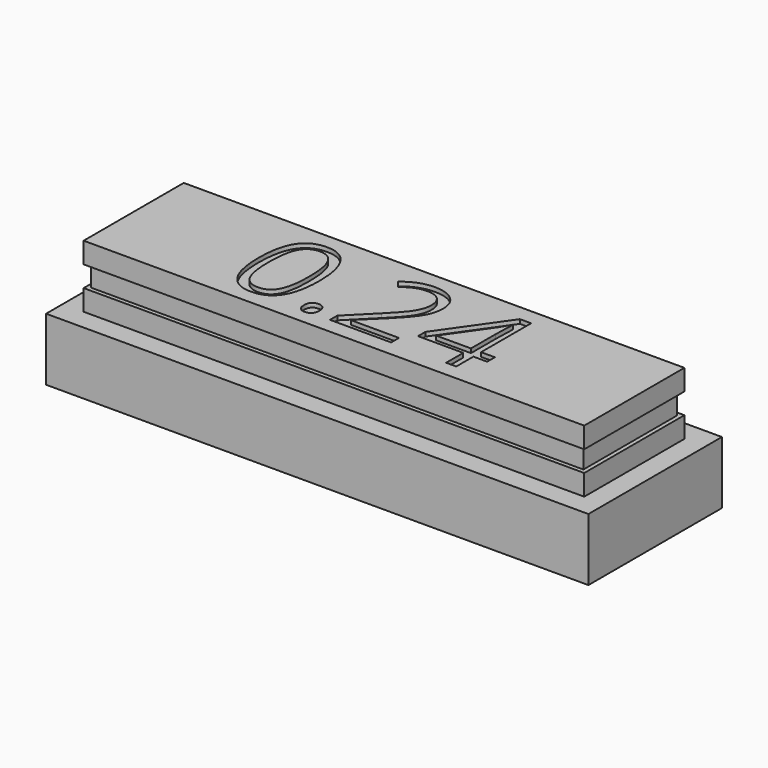
from build123d import *

# Parameters (mm, degrees)
F0_W         = 26
F0_H         = 8
F0_W_2       = 20
F0_H_2       = 2
F1_DEPTH     = 3
F2_W         = 24
F2_H         = 6
F3_DEPTH     = 3
F5_W         = 24
F5_H         = 6
F5_W_2       = 23.6
F5_H_2       = 5.6
F6_DEPTH     = 0.5
F7_W         = 19.52
F7_H         = 1.52
F8_DEPTH     = 3
F9_TEXT_SIZE = 6.25
F10_DEPTH    = 0.2


# Not quite as in the source:
# - Text() gives the source's letters only with a copy of the font that has no kerning and outlines rounded to 1/6400 em; it was checked with that copy


with BuildPart() as f1:
    # F0 (on Top) → F1 (new body)
    with BuildSketch(Plane.XY):
        Rectangle(F0_W, F0_H)
        Rectangle(F0_W_2, F0_H_2, mode=Mode.SUBTRACT)
    extrude(amount=F1_DEPTH)


with BuildPart() as f3:
    # F2 (on face) → F3 (new body)
    with BuildSketch(Plane.XY.offset(3)):
        Rectangle(F2_W, F2_H)
    extrude(amount=F3_DEPTH)

    # F5 (on mid) → F6 (cut, symmetric)
    with BuildSketch(Plane.XY.offset(4.5)):
        Rectangle(F5_W, F5_H)
        Rectangle(F5_W_2, F5_H_2, mode=Mode.SUBTRACT)
    extrude(amount=F6_DEPTH, both=True, mode=Mode.SUBTRACT)

    # F7 (on face) → F8 (join, through all)
    with BuildSketch(Plane(origin=(0, 0, 3), x_dir=(1, 0, 0), z_dir=(0, 0, -1))):
        Rectangle(F7_W, F7_H)
    extrude(amount=F8_DEPTH)

    # F9 (on face) → F10 (cut)
    with BuildSketch(Plane.XY.offset(6)):
        with Locations((-6.3315429688, -2.25)):
            Text('0.24', F9_TEXT_SIZE, font='Open Sans', text_align=(TextAlign.LEFT, TextAlign.BOTTOM))
    extrude(amount=-F10_DEPTH, mode=Mode.SUBTRACT)


solid = Compound([f1.part, f3.part])
